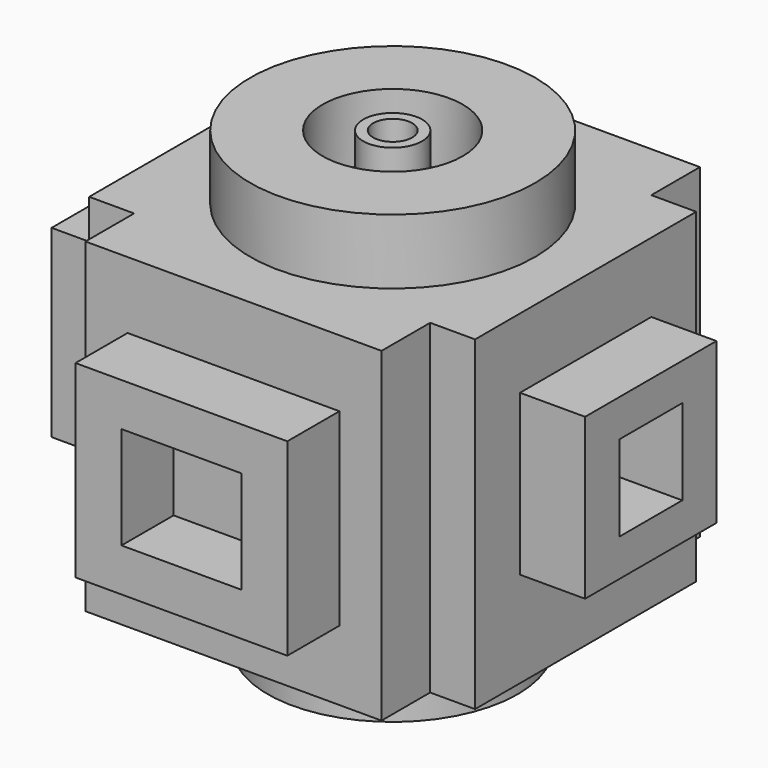
from build123d import *

# Parameters (mm, degrees)
F0_W      = 115.5085265636
F0_H      = 107.8471690416
F0_W_2    = 17.5325423479
F0_H_2    = 23.7205028534
F1_DEPTH  = 127
F2_R      = 55.6100218135
F2_R_2    = 41.4969022391
F2_R_3    = 27.3255706414
F2_R_4    = 11.4895056952
F2_R_5    = 7.610471178
F3_DEPTH  = 25.4
F4_W      = 64.0326142311
F4_H      = 62.4924302101
F4_W_2    = 30.7222977281
F4_H_2    = 33.4180146456
F5_DEPTH  = 25.4
F6_W      = 61.6823285818
F6_H      = 65.940104425
F6_W_2    = 35.1780280471
F6_H_2    = 32.1564599872
F7_DEPTH  = 25.4
F8_W      = 82.6514363289
F8_H      = 73.6512206495
F8_W_2    = 46.7445999384
F8_H_2    = 39.9785265326
F9_DEPTH  = 25.4
F10_W     = 81.0015127063
F10_H     = 71.895327419
F10_W_2   = 39.0375070274
F10_H_2   = 38.2135286927
F11_DEPTH = 25.4
F12_R     = 48.8134428036
F12_R_2   = 30.6319229548
F12_R_3   = 9.5593039908
F13_DEPTH = 25.4


with BuildPart() as f1:
    # F0 (on Top) → F1 (new body)
    with BuildSketch(Plane.XY):
        Rectangle(F0_W, F0_H)
        with Locations((-66.5205344558, 0)):
            Rectangle(F0_W_2, F0_H)
        with Locations((0, 65.7838359475)):
            Rectangle(F0_W, F0_H_2)
        with Locations((66.5205344558, 0)):
            Rectangle(F0_W_2, F0_H)
        with Locations((0, -65.7838359475)):
            Rectangle(F0_W, F0_H_2)
    extrude(amount=F1_DEPTH)

    # F2 (on face) → F3 (join)
    with BuildSketch(Plane.XY.offset(127)):
        Circle(F2_R)
        Circle(F2_R_2, mode=Mode.SUBTRACT)
        Circle(F2_R_2)
        Circle(F2_R_3, mode=Mode.SUBTRACT)
        Circle(F2_R_4)
        Circle(F2_R_5, mode=Mode.SUBTRACT)
    extrude(amount=F3_DEPTH)

    # F4 (on face) → F5 (join)
    with BuildSketch(Plane.YZ.offset(75.2868056297)):
        with Locations((0, 68.5164183378)):
            Rectangle(F4_W, F4_H)
        with Locations((0, 68.5164183378)):
            Rectangle(F4_W_2, F4_H_2, mode=Mode.SUBTRACT)
    extrude(amount=F5_DEPTH)

    # F6 (on face) → F7 (join)
    with BuildSketch(Plane(origin=(0, 77.6440873742, 0), x_dir=(-1, 0, 0), z_dir=(0, 1, 0))):
        with Locations((0, 61.1903108656)):
            Rectangle(F6_W, F6_H)
        with Locations((0, 61.1903108656)):
            Rectangle(F6_W_2, F6_H_2, mode=Mode.SUBTRACT)
    extrude(amount=F7_DEPTH)

    # F8 (on face) → F9 (join)
    with BuildSketch(Plane.XZ.offset(77.6440873742)):
        with Locations((0, 64.0937909484)):
            Rectangle(F8_W, F8_H)
        with Locations((0, 64.0937909484)):
            Rectangle(F8_W_2, F8_H_2, mode=Mode.SUBTRACT)
    extrude(amount=F9_DEPTH)

    # F10 (on face) → F11 (join)
    with BuildSketch(Plane(origin=(-75.2868056297, 0, 0), x_dir=(0, -1, 0), z_dir=(-1, 0, 0))):
        with Locations((0, 66.6888132691)):
            Rectangle(F10_W, F10_H)
        with Locations((0, 66.6888132691)):
            Rectangle(F10_W_2, F10_H_2, mode=Mode.SUBTRACT)
    extrude(amount=F11_DEPTH)

    # F12 (on face) → F13 (join)
    with BuildSketch(Plane(origin=(0, 0, 0), x_dir=(1, 0, 0), z_dir=(0, 0, -1))):
        Circle(F12_R)
        Circle(F12_R_2, mode=Mode.SUBTRACT)
        Circle(F12_R_3)
    extrude(amount=F13_DEPTH)


solid = f1.part
